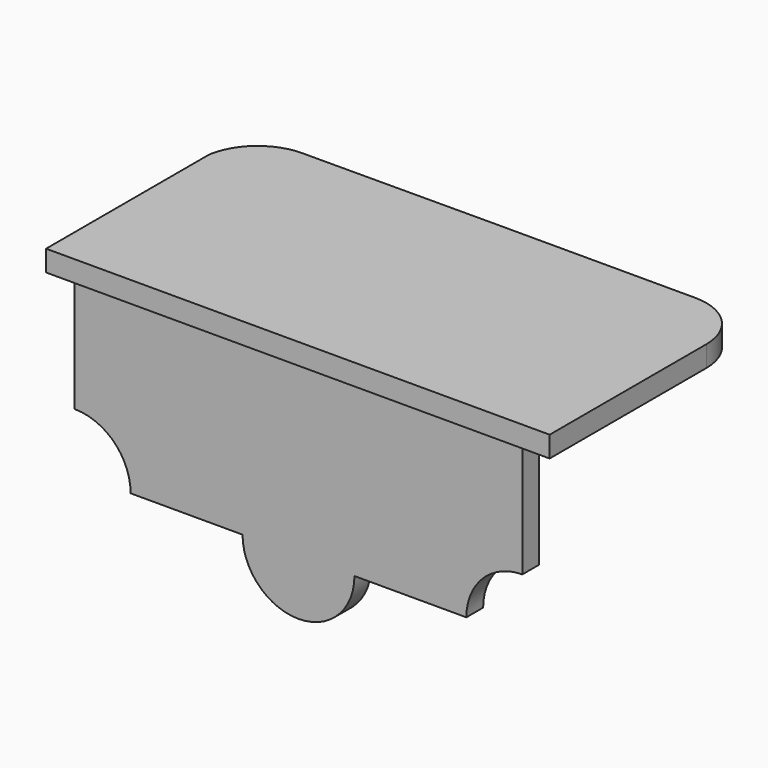
from build123d import *

# Parameters (mm, degrees)
F1_DEPTH = 9.525
F4_DEPTH = 76.2
F6_DEPTH = 9.525
F9_DEPTH = 25.4


# Not quite as in the source:
# - a feature of the source that left no trace in its solid (it failed there, or was rolled back) is left out


with BuildPart() as f1:
    # F0 (on Top) → F1 (new body)
    with BuildSketch(Plane.XY):
        with BuildLine():
            Line((0.2017877996, -54.3629787627), (0, 59.9370212373))
            Line((0, 59.9370212373), (-89.1012323912, 59.6224176037))
            ThreePointArc((-89.1012323912, 59.6224176037), (-105.5400958188, 53.5090257564), (-114.0982122004, 38.1999292884))
            Line((-114.0982122004, 38.1999292884), (-114.0982122004, -54.3629787627))
            Line((-114.0982122004, -54.3629787627), (0.2017877996, -54.3629787627))
        make_face()
        with BuildLine():
            Line((89.1017877996, 59.9370212373), (0, 59.9370212373))
            Line((0, 59.9370212373), (0.2017877996, -54.3629787627))
            Line((0.2017877996, -54.3629787627), (114.5017877996, -54.3629787627))
            Line((114.5017877996, -54.3629787627), (114.5017877996, 34.5370212373))
            ThreePointArc((114.5017877996, 34.5370212373), (107.0623000417, 52.4975334794), (89.1017877996, 59.9370212373))
        make_face()
    extrude(amount=F1_DEPTH)

    # F3 (on face) → F4 (join)
    with BuildSketch(Plane(origin=(0, 0, 0), x_dir=(1, 0, 0), z_dir=(0, 0, -1))):
        Polygon((4.8055368662, 44.1943933845), (0.0430368662, 44.1943933845), (0.0430368662, -43.7603956342), (4.8055368662, -43.7603956342), (4.8055368662, -34.2353956342), align=None)
        Polygon((0.0430368662, 44.1943933845), (-4.7194631338, 44.1943933845), (-4.7194631338, -34.2353956342), (-4.7194631338, -43.7603956342), (0.0430368662, -43.7603956342), align=None)
    extrude(amount=F4_DEPTH)

    # F8 (on face) → F9 (cut)
    with BuildSketch(Plane.YZ.offset(4.8055368662)):
        with BuildLine():
            Line((43.7603956342, -76.2), (43.7603956342, -12.7))
            ThreePointArc((43.7603956342, -12.7), (-1.6060003551, -32.6070556012), (-25.1443933845, -76.2))
            Line((-25.1443933845, -76.2), (43.7603956342, -76.2))
        make_face()
    extrude(amount=-F9_DEPTH, mode=Mode.SUBTRACT)


with BuildPart() as f6:
    # F5 (on face) → F6 (new body)
    with BuildSketch(Plane.XZ.offset(44.1943933845)):
        with BuildLine():
            Line((101.575226661, 0), (-101.624773339, 0))
            Line((-101.624773339, 0), (-101.624773339, -50.8))
            ThreePointArc((-101.624773339, -50.8), (-83.6642610969, -58.2394877579), (-76.224773339, -76.2))
            Line((-76.224773339, -76.2), (-25.424773339, -76.2))
            ThreePointArc((-25.424773339, -76.2), (-0.024773339, -101.6), (25.375226661, -76.2))
            Line((25.375226661, -76.2), (76.175226661, -76.2))
            ThreePointArc((76.175226661, -76.2), (83.6147144189, -58.2394877579), (101.575226661, -50.8))
            Line((101.575226661, -50.8), (101.575226661, 0))
        make_face()
    extrude(amount=F6_DEPTH)


solid = Compound([f1.part, f6.part])
